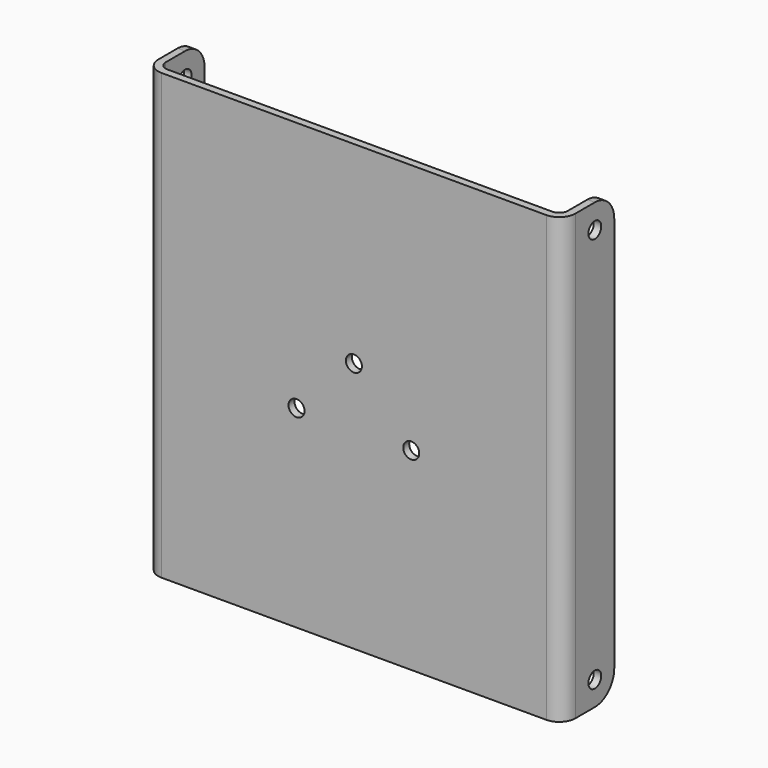
from build123d import *

# Parameters (mm, degrees)
F1_DEPTH = 101.6
F2_R     = 3.69316
F3_R     = 1.98374
F4_R     = 1.8288
F5_DEPTH = 95.37192
F6_R     = 5.55625
F7_R     = 1.8288
F8_DEPTH = 1.70942


with BuildPart() as f1:
    # F0 (on Top) → F1 (new body)
    with BuildSketch(Plane.XY):
        Polygon((0, 13.09624), (0, 0), (-91.95308, 0), (-91.95308, 13.09624), (-93.6625, 13.09624), (-93.6625, -1.70942), (1.70942, -1.70942), (1.70942, 13.09624), align=None)
    extrude(amount=F1_DEPTH)

    # F2
    f2_edges = [f1.edges().sort_by_distance(p)[0] for p in [
        (1.70942, -1.70942, 50.8),
        (-93.6625, -1.70942, 50.8),
    ]]
    fillet(f2_edges, radius=F2_R)

    # F3
    f3_edges = [f1.edges().sort_by_distance(p)[0] for p in [
        (0, 0, 50.8),
        (-91.95308, 0, 50.8),
    ]]
    fillet(f3_edges, radius=F3_R)

    # F4 (on face) → F5 (cut, through all)
    with BuildSketch(Plane.YZ.offset(1.70942)):
        with Locations((7.53999, 96.04375)):
            Circle(F4_R)
        with Locations((7.53999, 5.55625)):
            Circle(F4_R)
    extrude(amount=-F5_DEPTH, mode=Mode.SUBTRACT)

    # F6
    f6_edges = [f1.edges().sort_by_distance(p)[0] for p in [
        (-92.80779, 13.09624, 101.6),
        (-92.80779, 13.09624, 0),
        (0.85471, 13.09624, 0),
        (0.85471, 13.09624, 101.6),
    ]]
    fillet(f6_edges, radius=F6_R)

    # F7 (on face) → F8 (cut, through all)
    with BuildSketch(Plane(origin=(0, 0, 0), x_dir=(-1, 0, 0), z_dir=(0, 1, 0))):
        with Locations((59.0904203, 44.1744082526)):
            Circle(F7_R)
        with Locations((45.97654, 57.4255917474)):
            Circle(F7_R)
        with Locations((32.8626597, 44.1744082526)):
            Circle(F7_R)
    extrude(amount=-F8_DEPTH, mode=Mode.SUBTRACT)


solid = f1.part
